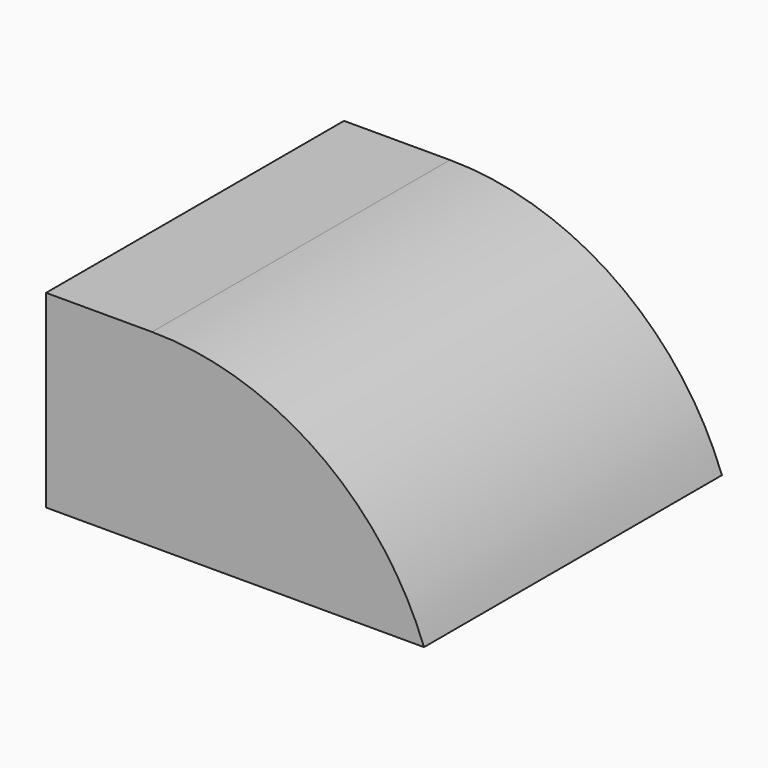
from build123d import *

# Parameters (mm, degrees)
F0_W        = 132.8576132655
F0_H        = 130.9104263783
F1_DEPTH    = 66.4626900107
F2_T1_DEPTH = 608.9647723724


# Not quite as in the source:
# - a fillet or chamfer that OpenCascade refuses, or shapes differently, is made with other operations: its cross-section is extruded or revolved along the edge and cut away or added


with BuildPart() as f1:
    # F0 (on Top) → F1 (new body)
    with BuildSketch(Plane.XY):
        with Locations((-0.6001107395, 0.1519322395)):
            Rectangle(F0_W, F0_H)
    extrude(amount=F1_DEPTH)

    # F2: fillet of radius 102.0025481231 on 1 edges, made by hand

    # F2_s2 → F2_t1 (cut)
    with BuildSketch(Plane.XZ.offset(-304.6343184257)):
        with BuildLine():
            ThreePointArc((65.8286958933, 0), (28.4388011633, 48.2147713447), (-29.7821733055, 66.4626900107))
            Line((-29.7821733055, 66.4626900107), (65.8286958933, 66.4626900107))
            Line((65.8286958933, 66.4626900107), (65.8286958933, 0))
        make_face()
    extrude(amount=F2_T1_DEPTH, mode=Mode.SUBTRACT)


solid = f1.part
